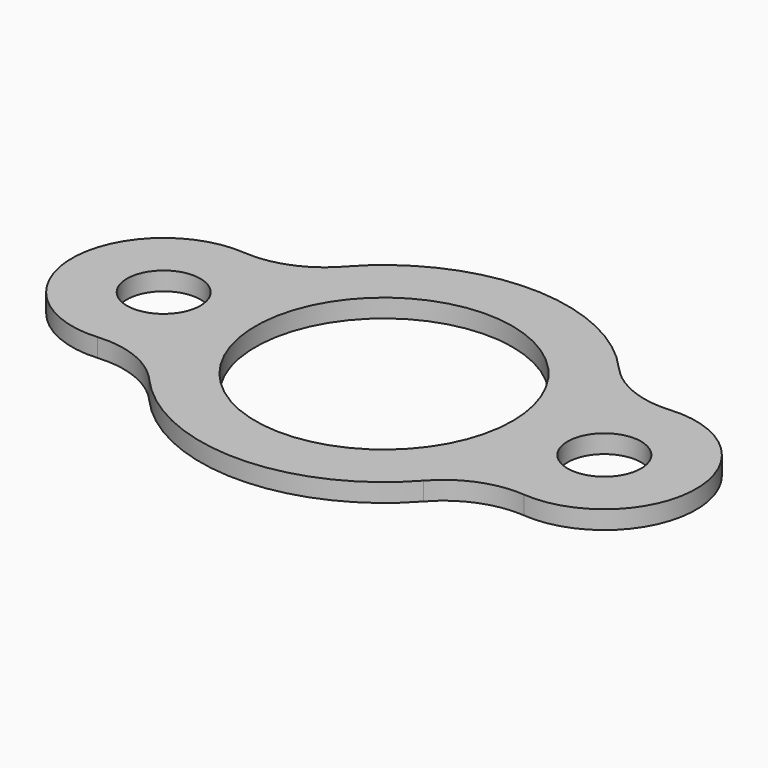
from build123d import *

# Parameters (mm, degrees)
F0_R     = 12.7
F0_R_2   = 44.45
F1_DEPTH = 6.35
F2_R     = 31.75


# Not quite as in the source:
# - a feature names something its author has since deleted; it is built from what else it names


with BuildPart() as f1:
    # F0 (on Top) → F1 (new body)
    with BuildSketch(Plane.XY):
        with BuildLine():
            ThreePointArc((-57.94375, 25.976370723), (-107.95, 0), (-57.94375, -25.976370723))
            ThreePointArc((-57.94375, -25.976370723), (0, -63.5), (57.94375, -25.976370723))
            ThreePointArc((57.94375, -25.976370723), (107.95, 0), (57.94375, 25.976370723))
            ThreePointArc((57.94375, 25.976370723), (0, 63.5), (-57.94375, 25.976370723))
        make_face()
        with Locations((-76.2, 0)):
            Circle(F0_R, mode=Mode.SUBTRACT)
        Circle(F0_R_2, mode=Mode.SUBTRACT)
        with Locations((76.2, 0)):
            Circle(F0_R, mode=Mode.SUBTRACT)
    extrude(amount=F1_DEPTH)

    # F2
    f2_edges = [f1.edges().sort_by_distance(p)[0] for p in [
        (-57.94375, -25.976371, 3.175),
        (57.94375, -25.976371, 3.175),
        (-57.94375, 25.976371, 3.175),
        (57.94375, 25.976371, 3.175),
    ]]
    fillet(f2_edges, radius=F2_R)


solid = f1.part
